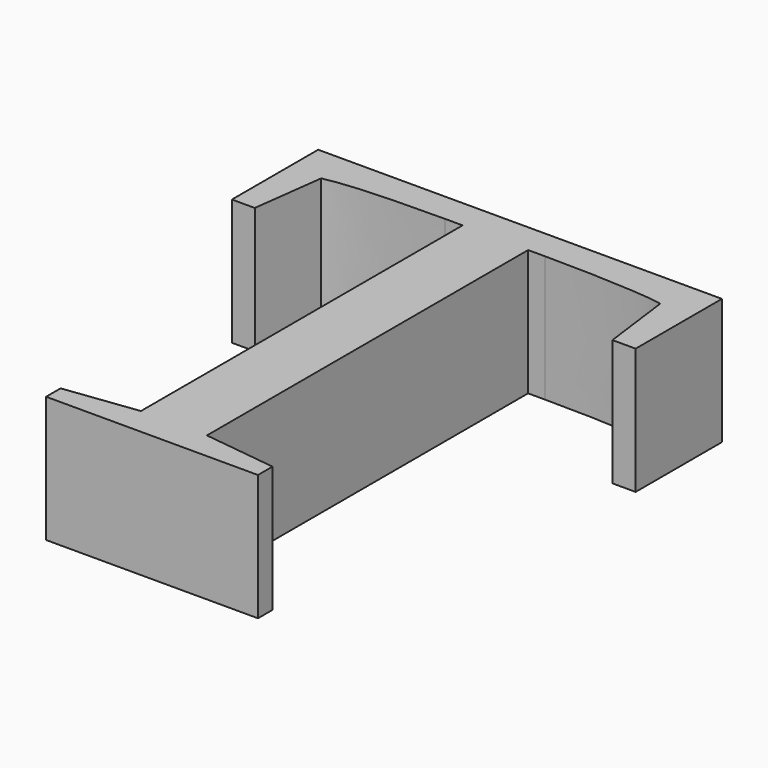
from build123d import *

# Parameters (mm, degrees)
F0_TEXT_SIZE = 141.1111111111
F1_DEPTH     = 25.4


# Not quite as in the source:
# - Text() gives the source's letters only with a copy of the font that has no kerning and outlines rounded to 1/6400 em; it was checked with that copy


with BuildPart() as f1:
    # F0 (on Top) → F1 (new body)
    with BuildSketch(Plane.XY):
        with Locations((-38.6198817054, -55.5532158662)):
            Text('T', F0_TEXT_SIZE, font='Tinos', text_align=(TextAlign.LEFT, TextAlign.BOTTOM))
    extrude(amount=F1_DEPTH)


solid = f1.part
